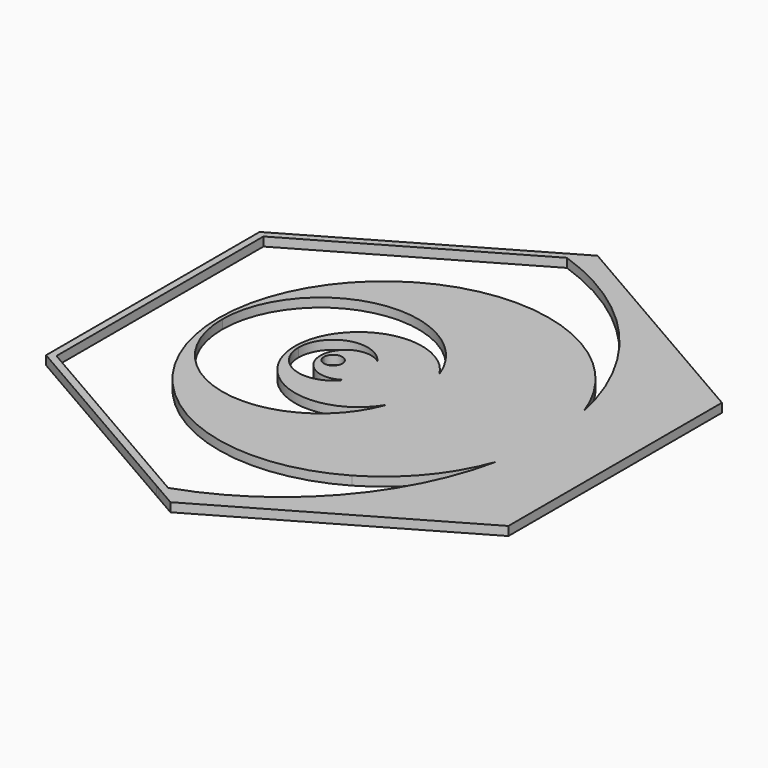
from build123d import *

# Parameters (mm, degrees)
F1_DEPTH = 2


# Not quite as in the source:
# - a feature names something its author has since deleted; it is built from what else it names


with BuildPart() as f1:
    # F0 (on Top) → F1 (new body)
    with BuildSketch(Plane.XY):
        with BuildLine():
            ThreePointArc((57.9139967595, 12.2722697167), (51.4568761016, 23.699090905), (41.428568188, 32.1666578549))
            ThreePointArc((41.428568188, 32.1666578549), (4.2857110581, 32.1666578623), (-14.2857175262, 2.97e-08))
            ThreePointArc((-14.2857175262, 2.97e-08), (-13.7653951877, 4.8492709465), (-12.2281175262, 9.477763266))
            ThreePointArc((-12.2281175262, 9.477763266), (9.6494218868, 33.857930499), (42.2568983073, 30.7319480028))
            ThreePointArc((42.2568983073, 30.7319480028), (54.3309771484, 18.1714285714), (59.1716666402, 1.434709852))
            ThreePointArc((59.1716666402, 1.434709852), (59.1929135394, 0.7174947657), (59.1999967595, 0))
            ThreePointArc((59.1999967595, 0), (58.8776189941, 6.1697325712), (57.9139967595, 12.2722697167))
        make_face()
        with BuildLine():
            ThreePointArc((-12.2281175262, -9.477763266), (-13.765395194, -4.8492709174), (-14.2857175262, 2.97e-08))
            ThreePointArc((-14.2857175262, 2.97e-08), (4.2857110323, -32.1666578474), (41.428568188, -32.1666578549))
            ThreePointArc((41.428568188, -32.1666578549), (51.4568761016, -23.699090905), (57.9139967595, -12.2722697167))
            ThreePointArc((57.9139967595, -12.2722697167), (58.8776189941, -6.1697325712), (59.1999967595, 0))
            ThreePointArc((59.1999967595, 0), (59.1929135394, -0.7174947657), (59.1716666402, -1.434709852))
            ThreePointArc((59.1716666402, -1.434709852), (54.3309771484, -18.1714285714), (42.2568983073, -30.7319480028))
            ThreePointArc((42.2568983073, -30.7319480028), (9.6494218868, -33.857930499), (-12.2281175262, -9.477763266))
        make_face()
        with BuildLine():
            ThreePointArc((-12.2281175262, 9.477763266), (-13.7653951877, 4.8492709465), (-14.2857175262, 2.97e-08))
            ThreePointArc((-14.2857175262, 2.97e-08), (-13.765395194, -4.8492709174), (-12.2281175262, -9.477763266))
            ThreePointArc((-12.2281175262, -9.477763266), (-13.1699457223, -4.7804170624), (-13.4857175262, 2.704e-07))
            ThreePointArc((-13.4857175262, 2.704e-07), (-13.1699456867, 4.7804173304), (-12.2281175262, 9.477763266))
        make_face()
        with BuildLine():
            ThreePointArc((19.1553909751, 56.0152735639), (44.3089741522, 39.2600881611), (57.9139967595, 12.2722697167))
            ThreePointArc((57.9139967595, 12.2722697167), (59.4747834067, 6.2241465278), (59.9999967595, 0))
            ThreePointArc((59.9999967595, 0), (49.011359006, 34.6104950953), (20.070451068, 56.5435837549))
            Line((20.070451068, 56.5435837549), (19.1553909751, 56.0152735639))
        make_face()
        with BuildLine():
            ThreePointArc((59.9999967595, 0), (59.4747834067, 6.2241465278), (57.9139967595, 12.2722697167))
            ThreePointArc((57.9139967595, 12.2722697167), (58.8776189941, 6.1697325712), (59.1999967595, 0))
            ThreePointArc((59.1999967595, 0), (58.8776189941, -6.1697325712), (57.9139967595, -12.2722697167))
            ThreePointArc((57.9139967595, -12.2722697167), (59.4747834067, -6.2241465278), (59.9999967595, 0))
        make_face()
        with BuildLine():
            ThreePointArc((42.2568983073, 30.7319480028), (9.6494218868, 33.857930499), (-12.2281175262, 9.477763266))
            ThreePointArc((-12.2281175262, 9.477763266), (13.4206962629, 22.3368205217), (31.428568188, 0))
            ThreePointArc((31.428568188, 0), (13.4206962629, -22.3368205217), (-12.2281175262, -9.477763266))
            ThreePointArc((-12.2281175262, -9.477763266), (9.6494218868, -33.857930499), (42.2568983073, -30.7319480028))
            ThreePointArc((42.2568983073, -30.7319480028), (54.3309771484, -18.1714285714), (59.1716666402, -1.434709852))
            ThreePointArc((59.1716666402, -1.434709852), (59.1929135394, -0.7174947657), (59.1999967595, 0))
            ThreePointArc((59.1999967595, 0), (59.1929135394, 0.7174947657), (59.1716666402, 1.434709852))
            ThreePointArc((59.1716666402, 1.434709852), (54.3309771484, 18.1714285714), (42.2568983073, 30.7319480028))
        make_face()
        with BuildLine():
            ThreePointArc((31.428568188, 0), (13.4206962629, 22.3368205217), (-12.2281175262, 9.477763266))
            ThreePointArc((-12.2281175262, 9.477763266), (-13.1699456867, 4.7804173304), (-13.4857175262, 2.704e-07))
            ThreePointArc((-13.4857175262, 2.704e-07), (4.7908132688, 21.7307276329), (29.332568188, 7.4493287138))
            ThreePointArc((29.332568188, 7.4493287138), (30.8945884868, 3.8692930325), (31.428568188, 0))
        make_face()
        with BuildLine():
            ThreePointArc((-13.4857175262, 2.704e-07), (-13.1699457223, -4.7804170624), (-12.2281175262, -9.477763266))
            ThreePointArc((-12.2281175262, -9.477763266), (13.4206962629, -22.3368205217), (31.428568188, 0))
            ThreePointArc((31.428568188, 0), (30.8945884868, -3.8692930325), (29.332568188, -7.4493287138))
            ThreePointArc((29.332568188, -7.4493287138), (4.7908130024, -21.7307275866), (-13.4857175262, 2.704e-07))
        make_face()
        with BuildLine():
            ThreePointArc((20.070451068, -56.5435837549), (49.011359006, -34.6104950953), (59.9999967595, 0))
            ThreePointArc((59.9999967595, 0), (59.4747834067, -6.2241465278), (57.9139967595, -12.2722697167))
            ThreePointArc((57.9139967595, -12.2722697167), (44.3089741522, -39.2600881611), (19.1553909751, -56.0152735639))
            Line((19.1553909751, -56.0152735639), (20.070451068, -56.5435837549))
        make_face()
        with BuildLine():
            ThreePointArc((20.070451068, 56.5435837549), (49.011359006, 34.6104950953), (59.9999967595, 0))
            ThreePointArc((59.9999967595, 0), (49.011359006, -34.6104950953), (20.070451068, -56.5435837549))
            Line((20.070451068, -56.5435837549), (22.8571396166, -58.1524791386))
            Line((22.8571396166, -58.1524791386), (73.2186638437, -29.0762395693))
            Line((73.2186638437, -29.0762395693), (73.2186638437, 29.0762395693))
            Line((73.2186638437, 29.0762395693), (22.8571396166, 58.1524791386))
            Line((22.8571396166, 58.1524791386), (20.070451068, 56.5435837549))
        make_face()
        with BuildLine():
            Line((-27.5043846104, 29.0762395693), (19.1553909751, 56.0152735639))
            ThreePointArc((19.1553909751, 56.0152735639), (18.1309499488, 56.3551997286), (17.1004817443, 56.6763920278))
            Line((17.1004817443, 56.6763920278), (-29.1043846104, 30))
            Line((-29.1043846104, 30), (-29.1043846104, -30))
            Line((-29.1043846104, -30), (17.1004817443, -56.6763920278))
            ThreePointArc((17.1004817443, -56.6763920278), (18.1309499488, -56.3551997286), (19.1553909751, -56.0152735639))
            Line((19.1553909751, -56.0152735639), (-27.5043846104, -29.0762395693))
            Line((-27.5043846104, -29.0762395693), (-27.5043846104, 29.0762395693))
        make_face()
        with BuildLine():
            ThreePointArc((17.1004817443, 56.6763920278), (18.1309499488, 56.3551997286), (19.1553909751, 56.0152735639))
            Line((19.1553909751, 56.0152735639), (20.070451068, 56.5435837549))
            ThreePointArc((20.070451068, 56.5435837549), (19.0610073309, 56.891808514), (18.0455263515, 57.2220137862))
            Line((18.0455263515, 57.2220137862), (17.1004817443, 56.6763920278))
        make_face()
        with BuildLine():
            ThreePointArc((29.332568188, -7.4493287138), (30.8945884868, -3.8692930325), (31.428568188, 0))
            ThreePointArc((31.428568188, 0), (30.8945884868, 3.8692930325), (29.332568188, 7.4493287138))
            ThreePointArc((29.332568188, 7.4493287138), (30.3021529406, 3.7806121953), (30.628568188, 0))
            ThreePointArc((30.628568188, 0), (30.3021529406, -3.7806121953), (29.332568188, -7.4493287138))
        make_face()
        with BuildLine():
            Line((22.8571396166, -58.1524791386), (20.070451068, -56.5435837549))
            ThreePointArc((20.070451068, -56.5435837549), (19.0610073309, -56.891808514), (18.0455263515, -57.2220137862))
            Line((18.0455263515, -57.2220137862), (22.8571396166, -60))
            Line((22.8571396166, -60), (74.8186638437, -30))
            Line((74.8186638437, -30), (74.8186638437, 30))
            Line((74.8186638437, 30), (22.8571396166, 60))
            Line((22.8571396166, 60), (18.0455263515, 57.2220137862))
            ThreePointArc((18.0455263515, 57.2220137862), (19.0610073309, 56.891808514), (20.070451068, 56.5435837549))
            Line((20.070451068, 56.5435837549), (22.8571396166, 58.1524791386))
            Line((22.8571396166, 58.1524791386), (73.2186638437, 29.0762395693))
            Line((73.2186638437, 29.0762395693), (73.2186638437, -29.0762395693))
            Line((73.2186638437, -29.0762395693), (22.8571396166, -58.1524791386))
        make_face()
        with BuildLine():
            ThreePointArc((18.0455263515, -57.2220137862), (19.0610073309, -56.891808514), (20.070451068, -56.5435837549))
            Line((20.070451068, -56.5435837549), (19.1553909751, -56.0152735639))
            ThreePointArc((19.1553909751, -56.0152735639), (18.1309499488, -56.3551997286), (17.1004817443, -56.6763920278))
            Line((17.1004817443, -56.6763920278), (18.0455263515, -57.2220137862))
        make_face()
        with BuildLine():
            ThreePointArc((30.628568188, 0), (30.3021529406, 3.7806121953), (29.332568188, 7.4493287138))
            ThreePointArc((29.332568188, 7.4493287138), (13.2735608698, 13.7517345845), (2.8571396166, 0))
            ThreePointArc((2.8571396166, 0), (3.3577591094, 2.8864214127), (4.8011396166, 5.4356764331))
            ThreePointArc((4.8011396166, 5.4356764331), (19.9202319053, 13.1966155216), (30.628568188, 0))
        make_face()
        with BuildLine():
            ThreePointArc((2.8571396166, 0), (13.2735608698, -13.7517345845), (29.332568188, -7.4493287138))
            ThreePointArc((29.332568188, -7.4493287138), (30.3021529406, -3.7806121953), (30.628568188, 0))
            ThreePointArc((30.628568188, 0), (19.9202319053, -13.1966155216), (4.8011396166, -5.4356764331))
            ThreePointArc((4.8011396166, -5.4356764331), (3.3577591094, -2.8864214127), (2.8571396166, 0))
        make_face()
        with BuildLine():
            ThreePointArc((4.8011396166, 5.4356764331), (3.3577591094, 2.8864214127), (2.8571396166, 0))
            ThreePointArc((2.8571396166, 0), (3.3577591094, -2.8864214127), (4.8011396166, -5.4356764331))
            ThreePointArc((4.8011396166, -5.4356764331), (3.9462383831, -2.7773780141), (3.6571396166, -2.26e-08))
            ThreePointArc((3.6571396166, -2.26e-08), (3.9462383784, 2.7773779919), (4.8011396166, 5.4356764331))
        make_face()
        with BuildLine():
            ThreePointArc((4.8011396166, -5.4356764331), (19.9202319053, -13.1966155216), (30.628568188, 0))
            ThreePointArc((30.628568188, 0), (19.9202319053, 13.1966155216), (4.8011396166, 5.4356764331))
            ThreePointArc((4.8011396166, 5.4356764331), (14.3149896007, 8.0708090786), (19.9999967595, 0))
            ThreePointArc((19.9999967595, 0), (14.3149896007, -8.0708090786), (4.8011396166, -5.4356764331))
        make_face()
        with BuildLine():
            ThreePointArc((19.9999967595, 0), (14.3149896007, 8.0708090786), (4.8011396166, 5.4356764331))
            ThreePointArc((4.8011396166, 5.4356764331), (3.9462383784, 2.7773779919), (3.6571396166, -2.26e-08))
            ThreePointArc((3.6571396166, -2.26e-08), (9.0240010942, 7.3900716595), (17.7119967595, 4.5731419646))
            ThreePointArc((17.7119967595, 4.5731419646), (19.3960846487, 2.5567836939), (19.9999967595, 0))
        make_face()
        with BuildLine():
            ThreePointArc((3.6571396166, -2.26e-08), (3.9462383831, -2.7773780141), (4.8011396166, -5.4356764331))
            ThreePointArc((4.8011396166, -5.4356764331), (14.3149896007, -8.0708090786), (19.9999967595, 0))
            ThreePointArc((19.9999967595, 0), (19.3960846487, -2.5567836939), (17.7119967595, -4.5731419646))
            ThreePointArc((17.7119967595, -4.5731419646), (9.0240011157, -7.3900716665), (3.6571396166, -2.26e-08))
        make_face()
        with BuildLine():
            ThreePointArc((17.7119967595, -4.5731419646), (19.3960846487, -2.5567836939), (19.9999967595, 0))
            ThreePointArc((19.9999967595, 0), (19.3960846487, 2.5567836939), (17.7119967595, 4.5731419646))
            ThreePointArc((17.7119967595, 4.5731419646), (18.818639851, 2.4045670831), (19.1999967595, 0))
            ThreePointArc((19.1999967595, 0), (18.818639851, -2.4045670831), (17.7119967595, -4.5731419646))
        make_face()
        with BuildLine():
            ThreePointArc((19.1999967595, 0), (18.818639851, 2.4045670831), (17.7119967595, 4.5731419646))
            ThreePointArc((17.7119967595, 4.5731419646), (11.7289273535, 5.1103736046), (8.5714253309, 4.8e-09))
            ThreePointArc((8.5714253309, 4.8e-09), (8.9714253321, 1.4579829532), (10.0594253309, 2.5077306759))
            ThreePointArc((10.0594253309, 2.5077306759), (15.5859088323, 4.7391655168), (19.1999967595, 0))
        make_face()
        with BuildLine():
            ThreePointArc((8.5714253309, 4.8e-09), (11.7289273492, -5.1103736024), (17.7119967595, -4.5731419646))
            ThreePointArc((17.7119967595, -4.5731419646), (18.818639851, -2.4045670831), (19.1999967595, 0))
            ThreePointArc((19.1999967595, 0), (15.5859088323, -4.7391655168), (10.0594253309, -2.5077306759))
            ThreePointArc((10.0594253309, -2.5077306759), (8.9714253297, -1.457982949), (8.5714253309, 4.8e-09))
        make_face()
        with BuildLine():
            ThreePointArc((10.0594253309, 2.5077306759), (8.9714253321, 1.4579829532), (8.5714253309, 4.8e-09))
            ThreePointArc((8.5714253309, 4.8e-09), (8.9714253297, -1.457982949), (10.0594253309, -2.5077306759))
            ThreePointArc((10.0594253309, -2.5077306759), (9.5465455326, -1.3001978026), (9.3714253309, -3.2e-08))
            ThreePointArc((9.3714253309, -3.2e-08), (9.5465455241, 1.3001977717), (10.0594253309, 2.5077306759))
        make_face()
        with BuildLine():
            ThreePointArc((10.0594253309, -2.5077306759), (15.5859088323, -4.7391655168), (19.1999967595, 0))
            ThreePointArc((19.1999967595, 0), (15.5859088323, 4.7391655168), (10.0594253309, 2.5077306759))
            ThreePointArc((10.0594253309, 2.5077306759), (12.8865511392, 2.4571428571), (14.2857110452, 0))
            ThreePointArc((14.2857110452, 0), (12.8865511392, -2.4571428571), (10.0594253309, -2.5077306759))
        make_face()
        with BuildLine():
            ThreePointArc((14.2857110452, 0), (12.8865511392, 2.4571428571), (10.0594253309, 2.5077306759))
            ThreePointArc((10.0594253309, 2.5077306759), (9.5465455241, 1.3001977717), (9.3714253309, -3.2e-08))
            ThreePointArc((9.3714253309, -3.2e-08), (9.5465455326, -1.3001978026), (10.0594253309, -2.5077306759))
            ThreePointArc((10.0594253309, -2.5077306759), (12.8865511392, -2.4571428571), (14.2857110452, 0))
        make_face()
        with BuildLine():
            ThreePointArc((13.4857110452, 0), (11.4285682041, -2.0571428571), (9.3714253309, -3.2e-08))
            ThreePointArc((9.3714253309, -3.2e-08), (11.428568172, 2.0571428571), (13.4857110452, 0))
        make_face(mode=Mode.SUBTRACT)
    extrude(amount=F1_DEPTH)


solid = f1.part
